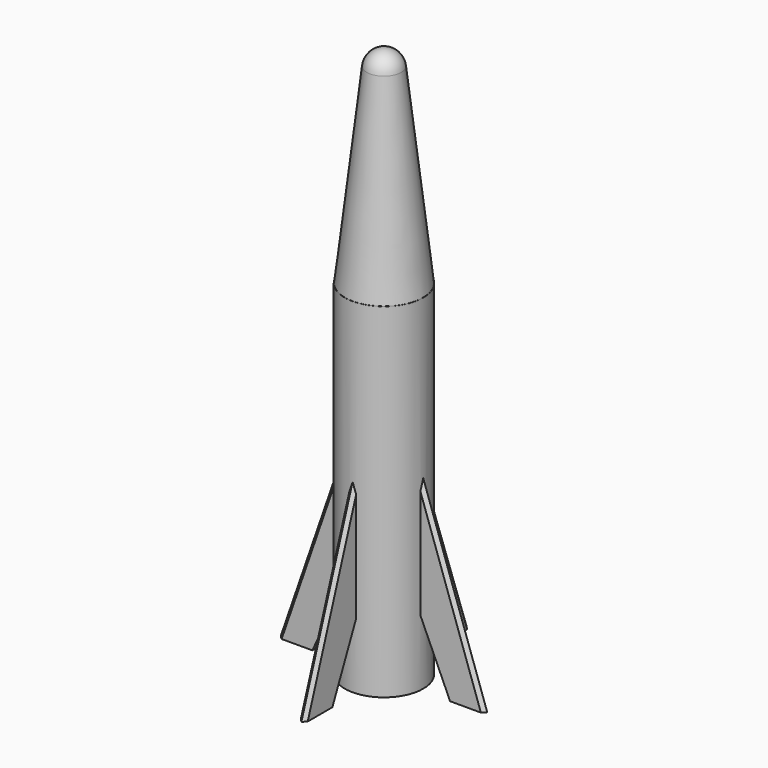
from build123d import *

# Parameters (mm, degrees)
F0_R            = 11.4
F0_R_2          = 8.9
F1_DEPTH        = 70
F7_DEPTH        = 1
F7_COPIES_COUNT = 4
F8_SIZE         = 0.9999
F2_R            = 11.4
F2_R_2          = 8.9
F9_DEPTH        = 30
F10_R           = 8.78
F11_DEPTH       = 8
F13_R           = 5
F13_R_2         = 3
F14_DEPTH       = 10
F15_R           = 5
F15_R_2         = 3
F16_DEPTH       = 10
F17_R           = 5.78
F18_DEPTH       = 50
F19_R           = 5


# Not quite as in the source:
# - a fillet or chamfer is up to 0.001 mm smaller than in the source, because OpenCascade refuses the exact size
# - a pattern or mirror of a feature is missing from the dataset's text; its kind, count and spacing are read off the source's solid


with BuildPart() as f1:
    # F0 (on Top) → F1 (new body)
    with BuildSketch(Plane.XY):
        Circle(F0_R)
        Circle(F0_R_2, mode=Mode.SUBTRACT)
    extrude(amount=F1_DEPTH)

    # F6 (on Front) → F7 (join, symmetric)
    with BuildSketch(Plane.XZ):
        Polygon((-30, 0), (-20, 0), (-11, 20), (-11, 55), align=None)
    f7 = extrude(amount=F7_DEPTH, both=True)

    # F7_copies: F7 ×4 about axis
    f7_copies_axis = Axis((0, 0, 0), (0, 0, 1))
    for i in range(1, F7_COPIES_COUNT):
        add(f7.rotate(f7_copies_axis, i * 360 / F7_COPIES_COUNT))

    # F8 (size 1 in the source; OpenCascade refuses exactly that, so slightly less here)
    f8_edges = [f1.edges().sort_by_distance(p)[0] for p in [
        (-20.678028, -1, 26.984656),
        (-20.678028, 1, 26.984656),
        (20.678028, -1, 26.984656),
        (20.678028, 1, 26.984656),
        (-1, 20.678028, 26.984656),
        (1, 20.678028, 26.984656),
        (1, -20.678028, 26.984656),
        (-1, -20.678028, 26.984656),
    ]]
    chamfer(f8_edges, length=F8_SIZE)

    # F2 (on face) → F9 (join)
    with BuildSketch(Plane.XY.offset(70)):
        Circle(F2_R)
        Circle(F2_R_2, mode=Mode.SUBTRACT)
    extrude(amount=F9_DEPTH)

    # F13 (on offset) → F14 (join)
    with BuildSketch(Plane.XY.offset(90)):
        with Locations((-13.0966598795, 7)):
            Circle(F13_R)
        with Locations((-13.0966598795, 7)):
            Circle(F13_R_2, mode=Mode.SUBTRACT)
    extrude(amount=-F14_DEPTH)

    # F15 (on Top) → F16 (join)
    with BuildSketch(Plane.XY):
        with Locations((-13.0966598795, 7)):
            Circle(F15_R)
        with Locations((-13.0966598795, 7)):
            Circle(F15_R_2, mode=Mode.SUBTRACT)
    extrude(amount=F16_DEPTH)


with BuildPart() as f5:
    # F4 (on Front) → F5 (revolve)
    with BuildSketch(Plane.XZ):
        with BuildLine():
            Line((-5, 155.5390949025), (-11.35, 100))
            Line((-11.35, 100), (0, 100))
            Line((0, 100), (0, 160))
            ThreePointArc((0, 160), (-3.3503609615, 158.7226734906), (-5, 155.5390949025))
        make_face()
    revolve(axis=Axis((0, 0, 130), (0, 0, -1)))

    # F10 (on face) → F11 (join)
    with BuildSketch(Plane(origin=(0, 0, 100), x_dir=(1, 0, 0), z_dir=(0, 0, -1))):
        Circle(F10_R)
    extrude(amount=F11_DEPTH)

    # F17 (on face) → F18 (cut)
    with BuildSketch(Plane(origin=(0, 0, 92), x_dir=(1, 0, 0), z_dir=(0, 0, -1))):
        Circle(F17_R)
    extrude(amount=-F18_DEPTH, mode=Mode.SUBTRACT)

    # F19
    f19_edges = [f5.edges().sort_by_distance(p)[0] for p in [
        (-5.78, 0, 142),
    ]]
    fillet(f19_edges, radius=F19_R)


solid = Compound([f1.part, f5.part])
